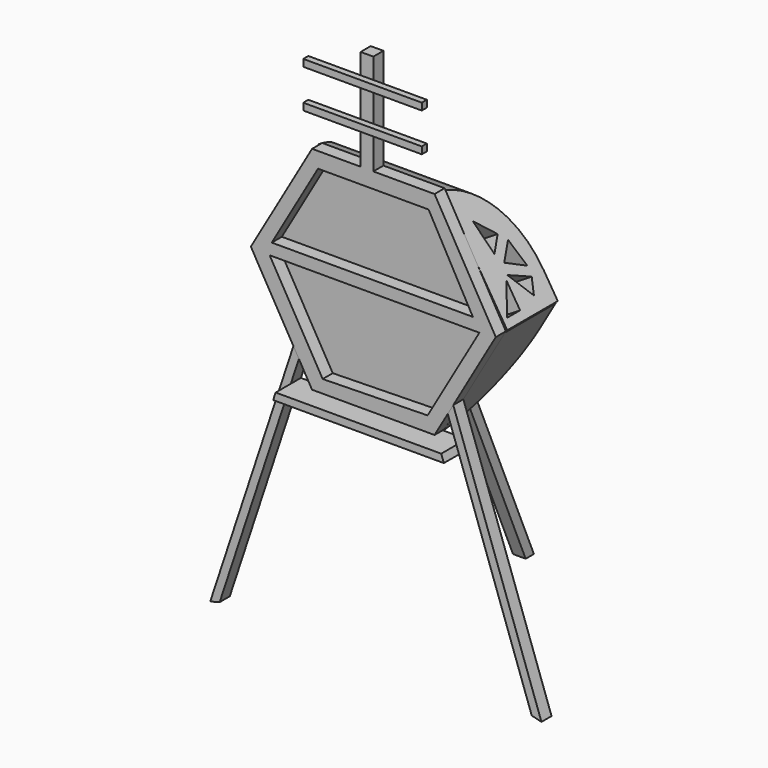
from build123d import *

# Parameters (mm, degrees)
F1_DEPTH    = 2.54
F2_DEPTH    = 6.35
F3_DEPTH    = 2.54
F5_DEPTH    = 12.7
F6_T1_DEPTH = 64.7979646342
F6_T3_DEPTH = 40.6008481475
F8_DEPTH    = 12.7
F9_T1_DEPTH = 104.7890423645
F12_DEPTH   = 2.54
F13_DEPTH   = 5.08
F14_DEPTH   = 5.08
F16_DEPTH   = 2.54
F17_W       = 2.5518944021
F17_H       = 2.54
F18_DEPTH   = 20.32
F19_W       = 10.5172891635
F19_H       = 1.4007464051
F19_W_2     = 10.7583077624
F19_W_3     = 2.5518944021
F19_H_2     = 1.397
F20_DEPTH   = 1.27


# Not quite as in the source:
# - a fillet or chamfer that OpenCascade refuses, or shapes differently, is made with other operations: its cross-section is extruded or revolved along the edge and cut away or added
# - a feature names something its author has since deleted; it is built from what else it names


with BuildPart() as f1:
    # F0 (on Front) → F1 (new body)
    with BuildSketch(Plane.XZ):
        Polygon((-12.3096870905, 24.5958147295), (12.3096870905, 24.5958147295), (14.9623812482, 29.1904157876), (16.0672812482, 31.1041587249), (24.619374181, 45.9168181956), (12.3096870905, 67.2378216616), (-12.3096870905, 67.2378216616), (-24.619374181, 45.9168181956), (-16.063203778, 31.0970963393), (-14.9623812482, 29.1904157876), align=None)
        Polygon((-20.4179584605, 47.9999661041), (-11.1165930793, 64.1104035241), (11.1165930793, 64.1104035241), (20.0077917219, 47.9999661041), (21.3189943773, 45.6241280226), (10.9129743139, 27.6003725681), (-10.1836063763, 27.1850443882), (-20.8387417213, 45.6241280226), (-21.3144036201, 46.4472775415), align=None, mode=Mode.SUBTRACT)
    extrude(amount=F1_DEPTH)

    # F0 (on Front) → F3 (join)
    with BuildSketch(Plane.XZ):
        Polygon((20.0077917219, 47.9999661041), (-20.4179584605, 47.9999661041), (-21.3144036201, 46.4472775415), (-20.8387417213, 45.6241280226), (21.3189943773, 45.6241280226), align=None)
    extrude(amount=F3_DEPTH)

    # F4 (on Front) → F5 (join)
    with BuildSketch(Plane.XZ):
        Polygon((-24.6073901653, 46.1928248405), (24.8951986432, 46.1928248405), (12.076173909, 66.8027698994), (-13.0007863045, 66.8027698994), align=None)
    extrude(amount=-F5_DEPTH)

    # F6: fillet of radius 16.51 on 1 edges, made by hand

    # F6_s2 → F6_t1 (cut)
    with BuildSketch(Plane.YZ.offset(-12.5608644411)):
        with BuildLine():
            ThreePointArc((12.7, 50.7383993857), (9.1415095645, 60.9774667261), (0, 66.8027698994))
            Line((0, 66.8027698994), (12.7, 66.8027698994))
            Line((12.7, 66.8027698994), (12.7, 50.7383993857))
        make_face()
    extrude(amount=F6_T1_DEPTH, mode=Mode.SUBTRACT)

    # F6_s4 → F6_t3 (cut)
    with BuildSketch(Plane.YZ.offset(-53.1617125886)):
        with BuildLine():
            ThreePointArc((12.7, 50.7383993857), (9.1415095645, 60.9774667261), (0, 66.8027698994))
            Line((0, 66.8027698994), (12.7, 66.8027698994))
            Line((12.7, 66.8027698994), (12.7, 50.7383993857))
        make_face()
    extrude(amount=F6_T3_DEPTH, mode=Mode.SUBTRACT)

    # F7 (on face) → F8 (join)
    with BuildSketch(Plane.XZ):
        Polygon((24.1872295737, 46.1016893387), (-24.1620466113, 46.1016893387), (-12.2359395027, 24.4347602129), (12.2312502936, 24.4347602129), (24.4206115603, 45.6104800105), align=None)
    extrude(amount=-F8_DEPTH)

    # F9: fillet of radius 16.51 on 1 edges, made by hand

    # F9_s2 → F9_t1 (cut)
    with BuildSketch(Plane.YZ.offset(-52.3968657869)):
        with BuildLine():
            ThreePointArc((0, 24.4347602129), (9.1415095645, 30.2600633862), (12.7, 40.4991307266))
            Line((12.7, 40.4991307266), (12.7, 24.4347602129))
            Line((12.7, 24.4347602129), (0, 24.4347602129))
        make_face()
    extrude(amount=F9_T1_DEPTH, mode=Mode.SUBTRACT)

    # F11 (on face) + F10 (on face) → F13 (cut)
    with BuildSketch(Plane(origin=(-38.4324941113, 0, 21.6434703373), x_dir=(0, -1, 0), z_dir=(-0.8713313746, 0, 0.4906950536))):
        Polygon((-4.3718703091, 39.4256524742), (-3.040788928, 45.6056557596), (-6.8525229581, 41.7865514755), align=None)
        Polygon((-5.4004341364, 37.411943078), (-8.3651151508, 40.1200354099), (-9.8777078092, 35.2593585849), align=None)
        Polygon((-5.0374120474, 35.5371125042), (-9.7567010671, 33.3913478812), (-8.3651151508, 30.7458732277), align=None)
        Polygon((-1.0033984436, 29.9311615527), (-4.3113664724, 35.0510440767), (-4.3113664724, 29.9311615527), align=None)
    with BuildSketch(Plane(origin=(38.6673789122, 0, 24.0504322194), x_dir=(0, 1, 0), z_dir=(0.8491479072, 0, 0.5281551209))):
        Polygon((6.8130241707, 40.0453992188), (3.022192046, 43.7935963273), (4.3540487314, 37.5584534102), align=None)
        Polygon((4.3540487314, 27.7913156897), (4.3540487314, 33.0006070435), (1.0958878556, 27.7913156897), align=None)
        Polygon((9.7206383943, 31.4991533315), (5.0109082768, 33.6494068058), (8.4560297574, 28.7292634302), align=None)
        Polygon((9.860817343, 33.3406813443), (8.3504421636, 38.4387634695), (5.5238169231, 35.5799859143), align=None)
    extrude(amount=-F13_DEPTH, dir=(-0.8713313746, 0, 0.4906950536), mode=Mode.SUBTRACT)

    # F10 (on face) → F14 (cut)
    with BuildSketch(Plane(origin=(38.6673789122, 0, 24.0504322194), x_dir=(0, 1, 0), z_dir=(0.8491479072, 0, 0.5281551209))):
        Polygon((9.860817343, 33.3406813443), (8.3504421636, 38.4387634695), (5.5238169231, 35.5799859143), align=None)
        Polygon((9.7206383943, 31.4991533315), (5.0109082768, 33.6494068058), (8.4560297574, 28.7292634302), align=None)
        Polygon((4.3540487314, 27.7913156897), (4.3540487314, 33.0006070435), (1.0958878556, 27.7913156897), align=None)
        Polygon((6.8130241707, 40.0453992188), (3.022192046, 43.7935963273), (4.3540487314, 37.5584534102), align=None)
    extrude(amount=-F14_DEPTH, mode=Mode.SUBTRACT)

    # F15 (on Right) → F16 (join)
    with BuildSketch(Plane.YZ):
        Polygon((37.8151386976, -16.8852526695), (12.8690572456, 40.6673364341), (10.8043896034, 40.6673364341), (35.7504710555, -16.8852526695), align=None)
    extrude(amount=-F16_DEPTH)

    # F17 (on face) → F18 (join)
    with BuildSketch(Plane.XY.offset(67.2378216616)):
        with Locations((-1.2759472011, -1.27)):
            Rectangle(F17_W, F17_H)
    extrude(amount=F18_DEPTH)

    # F19 (on face) → F20 (join)
    with BuildSketch(Plane.XZ.offset(2.54)):
        with Locations((-7.8105389839, 82.721490413)):
            Rectangle(F19_W, F19_H)
        with Locations((5.3791538812, 82.721490413)):
            Rectangle(F19_W_2, F19_H)
        with Locations((-1.2759472011, 82.721490413)):
            Rectangle(F19_W_3, F19_H)
        with Locations((-7.8105389839, 74.9725780115)):
            Rectangle(F19_W, F19_H_2)
        with Locations((-1.2759472011, 74.9725780115)):
            Rectangle(F19_W_3, F19_H_2)
        with Locations((5.3791538812, 74.9725780115)):
            Rectangle(F19_W_2, F19_H_2)
    extrude(amount=F20_DEPTH)


with BuildPart() as f2:
    # F0 (on Front) → F2 (new body)
    with BuildSketch(Plane.XZ):
        Polygon((17.2293611918, 22.7602638308), (16.6998734149, 24.2621239926), (-16.5899691079, 24.2621239926), (-17.085964367, 22.7602638308), align=None)
    extrude(amount=F2_DEPTH)


with BuildPart() as f12:
    # F0 (on Front) → F12 (new body)
    with BuildSketch(Plane.XZ):
        Polygon((-16.5899691079, 24.2621239926), (-14.9623812482, 29.1904157876), (-16.063203778, 31.0970963393), (-32.79035625, -19.5522666397), (-30.8930026501, -19.0470727638), (-17.085964367, 22.7602638308), align=None)
    extrude(amount=F12_DEPTH)


with BuildPart() as f12b:
    # F0 (on Front) → F12, piece 2 (new body)
    with BuildSketch(Plane.XZ):
        Polygon((16.0672812482, 31.1041587249), (14.9623812482, 29.1904157876), (16.6998734149, 24.2621239926), (17.2293611918, 22.7602638308), (31.85317493, -18.7193023163), (33.8026146141, -19.2010452842), align=None)
    extrude(amount=F12_DEPTH)


solid = Compound([f1.part, f2.part, f12.part, f12b.part])
